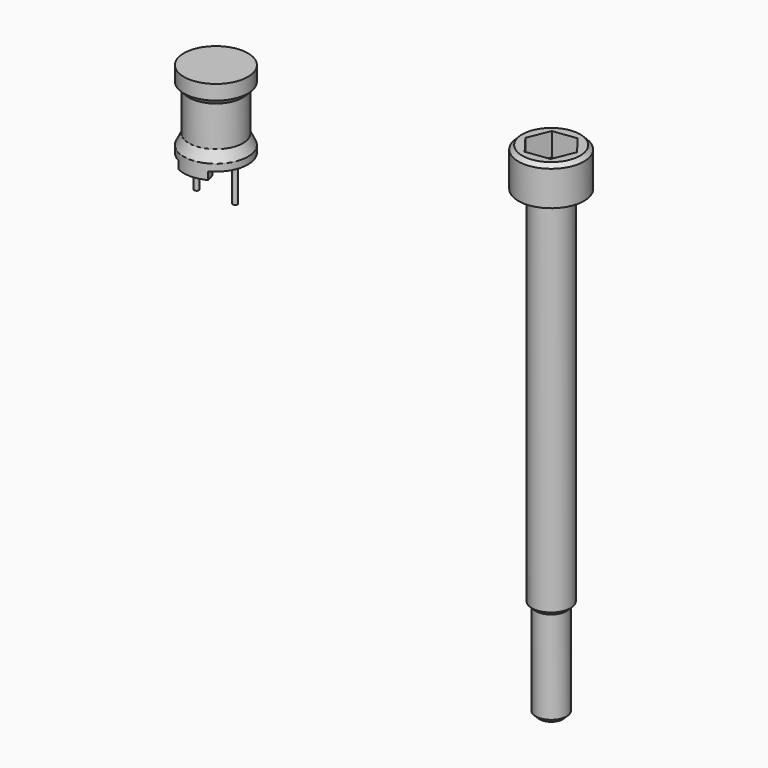
from build123d import *

# Parameters (mm, degrees)
F2_R     = 0.3
F3_DEPTH = 4
F4_DEPTH = 1
F7_DEPTH = 3
F8_SIZE  = 0.49999


# Not quite as in the source:
# - a fillet or chamfer is up to 0.001 mm smaller than in the source, because OpenCascade refuses the exact size


with BuildPart() as f1:
    # F0 (on Front) → F1 (revolve)
    with BuildSketch(Plane.XZ):
        Polygon((4.15, 0), (0, 0), (0, -11), (4.15, -11), (4.15, -9.1034269934), (3.5, -7.7787333211), (3.5, -2.5771334185), (4.15, -1.8965730066), align=None)
    revolve(axis=Axis((0, 0, -5.7281980938), (0, 0, -1)))

    # F2 (on face) → F3 (join)
    with BuildSketch(Plane(origin=(0, 0, -11), x_dir=(1, 0, 0), z_dir=(0, 0, -1))):
        with Locations((-2.5, 0)):
            Circle(F2_R)
        with Locations((2.5, 0)):
            Circle(F2_R)
    extrude(amount=F3_DEPTH)

    # F2 (on face) → F4 (cut)
    with BuildSketch(Plane(origin=(0, 0, -11), x_dir=(1, 0, 0), z_dir=(0, 0, -1))):
        with BuildLine():
            Line((-1.6264907317, 2.5791286025), (-1.9413472416, 3.6679246022))
            ThreePointArc((-1.9413472416, 3.6679246022), (-4.15, 0), (-1.9413472416, -3.6679246022))
            Line((-1.9413472416, -3.6679246022), (-1.6264907317, -2.5791286025))
            Line((-1.6264907317, -2.5791286025), (0, -2.5791286025))
            Line((0, -2.5791286025), (1.6264907317, -2.5791286025))
            Line((1.6264907317, -2.5791286025), (1.9413472416, -3.6679246022))
            ThreePointArc((1.9413472416, -3.6679246022), (3.555213851, -2.140783612), (4.15, 0))
            ThreePointArc((4.15, 0), (3.555213851, 2.140783612), (1.9413472416, 3.6679246022))
            Line((1.9413472416, 3.6679246022), (1.6264907317, 2.5791286025))
            Line((1.6264907317, 2.5791286025), (0, 2.5791286025))
            Line((0, 2.5791286025), (-1.6264907317, 2.5791286025))
        make_face()
        with Locations((-2.5, 0)):
            Circle(F2_R, mode=Mode.SUBTRACT)
        with Locations((2.5, 0)):
            Circle(F2_R, mode=Mode.SUBTRACT)
    extrude(amount=-F4_DEPTH, mode=Mode.SUBTRACT)


with BuildPart() as f5:
    # F0 (on Front) → F5 (revolve)
    with BuildSketch(Plane.XZ):
        Polygon((43.4252958298, 5), (43.4252958298, 0), (45.9252958298, 0), (47.6752958298, 0), (47.6752958298, 5), align=None)
        Polygon((45.9252958298, 0), (43.4252958298, 0), (43.4252958298, -60), (45.4252958298, -60), (45.4252958298, -47.5), (45.9252958298, -47.5), align=None)
    revolve(axis=Axis((43.4252958298, 0, -3.0905508995), (0, 0, -1)))

    # F6 (on face) → F7 (cut)
    with BuildSketch(Plane.XY.offset(5)):
        Polygon((46.4586920028, 0.3933412765), (44.6013503785, 2.8236687838), (41.5679542055, 2.4303275073), (40.3918996567, -0.3933412765), (42.2492412811, -2.8236687838), (45.2826374541, -2.4303275073), align=None)
    extrude(amount=-F7_DEPTH, mode=Mode.SUBTRACT)

    # F8 (size 0.5 in the source; OpenCascade refuses exactly that, so slightly less here)
    f8_edges = [f5.edges().sort_by_distance(p)[0] for p in [
        (39.175296, 0, 5),
        (40.925296, 0, 0),
        (40.925296, 0, -47.5),
        (41.425296, 0, -60),
    ]]
    chamfer(f8_edges, length=F8_SIZE)


solid = Compound([f1.part, f5.part])
